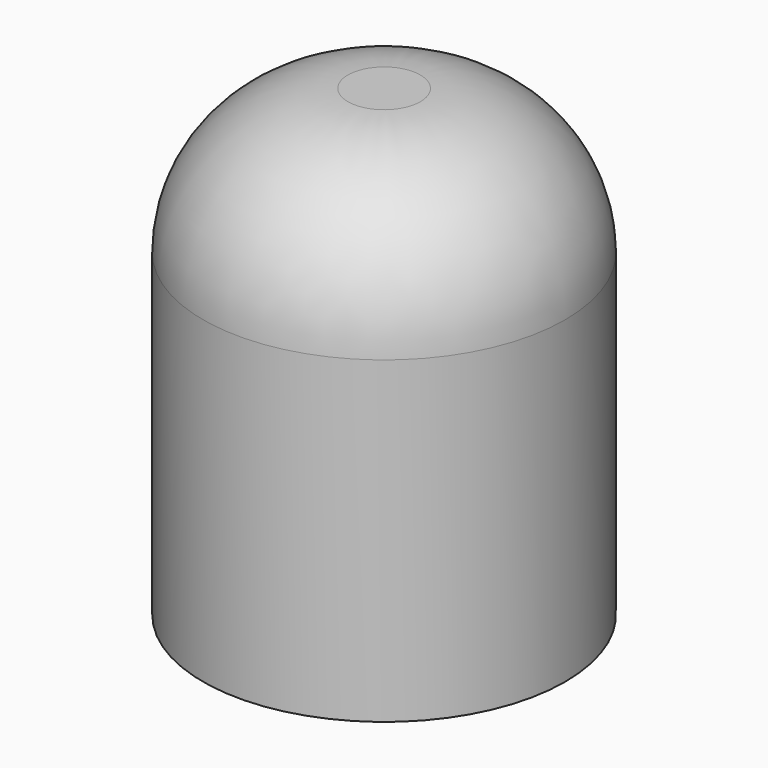
from build123d import *

# Parameters (mm, degrees)
F0_R     = 12.5
F1_DEPTH = 22
F3_DEPTH = 22
F4_R     = 12.5
F5_DEPTH = 10
F6_R     = 10
F8_DEPTH = 5
F9_R     = 4.99999


# Not quite as in the source:
# - a fillet or chamfer is up to 0.001 mm smaller than in the source, because OpenCascade refuses the exact size


with BuildPart() as f1:
    # F0 (on Top) → F1 (new body)
    with BuildSketch(Plane.XY):
        Circle(F0_R)
    extrude(amount=F1_DEPTH)

    # F2 (on face) → F3 (cut, through all)
    with BuildSketch(Plane(origin=(0, 0, 0), x_dir=(1, 0, 0), z_dir=(0, 0, -1))):
        Polygon((9, -5.1961524227), (9, 5.1961524227), (0, 10.3923048454), (-9, 5.1961524227), (-9, -5.1961524227), (0, -10.3923048454), align=None)
    extrude(amount=-F3_DEPTH, mode=Mode.SUBTRACT)

    # F4 (on face) → F5 (join)
    with BuildSketch(Plane.XY.offset(22)):
        Circle(F4_R)
    extrude(amount=F5_DEPTH)

    # F6
    f6_edges = [f1.edges().sort_by_distance(p)[0] for p in [
        (-12.5, 0, 32),
    ]]
    fillet(f6_edges, radius=F6_R)

    # F7 (on face) → F8 (cut)
    with BuildSketch(Plane(origin=(0, 0, 22), x_dir=(1, 0, 0), z_dir=(0, 0, -1))):
        with BuildLine():
            ThreePointArc((4.499999942, -7.7942286675), (7.7942286173, -4.500000029), (9, 0))
            ThreePointArc((9, 0), (7.7942286173, 4.500000029), (4.499999942, 7.7942286675))
            ThreePointArc((4.499999942, 7.7942286675), (-1.087e-07, 9), (-4.5000001303, 7.7942285588))
            ThreePointArc((-4.5000001303, 7.7942285588), (-7.7942286717, 4.4999999349), (-9, 0))
            ThreePointArc((-9, 0), (-7.7942286277, -4.500000011), (-4.499999978, -7.7942286468))
            ThreePointArc((-4.499999978, -7.7942286468), (-2.08e-08, -9), (4.499999942, -7.7942286675))
        make_face()
    extrude(amount=-F8_DEPTH, mode=Mode.SUBTRACT)

    # F9 (radius 5 in the source; OpenCascade refuses exactly that, so slightly less here)
    f9_edges = [f1.edges().sort_by_distance(p)[0] for p in [
        (-4.5, 7.794229, 27),
    ]]
    fillet(f9_edges, radius=F9_R)


solid = f1.part
